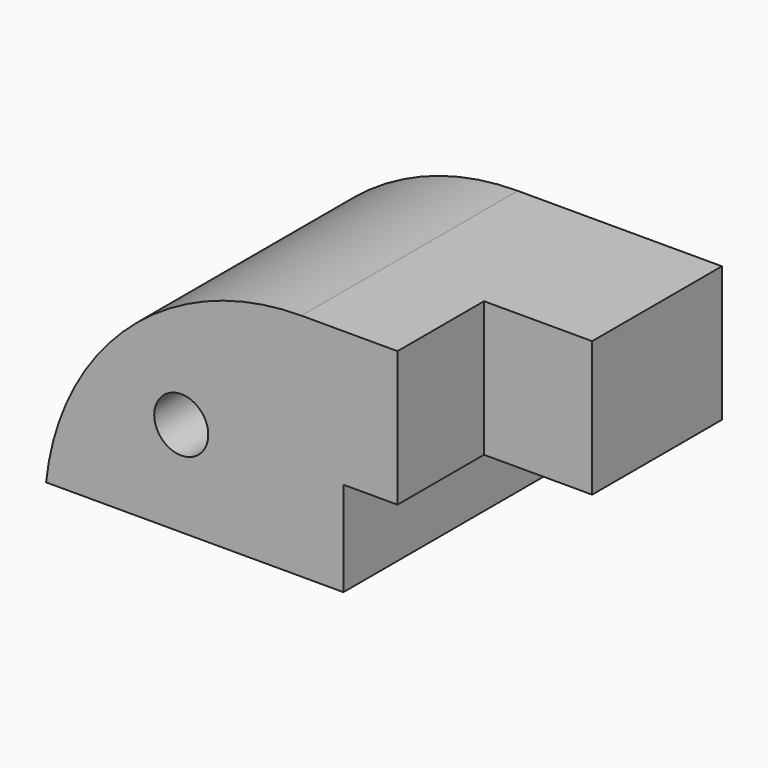
from build123d import *

# Parameters (mm, degrees)
F0_W         = 215.9
F0_H         = 127
F1_DEPTH     = 82.55
F2_W         = 76.2
F2_H         = 44.45
F3_DEPTH     = 127.001
F4_W         = 50.8
F4_H         = 37.5581905246
F5_DEPTH     = 82.551
F6_R         = 7.8160058593
F7_DEPTH     = 0.254
F8_R         = 12.7
F9_DEPTH     = 127.001
F10_T1_DEPTH = 699.3812649799
F11_DEPTH    = 107.95
F14_W        = 76.2
F14_H        = 44.45
F15_DEPTH    = 127.001
F13_W        = 50.8
F13_H        = 63.5
F16_DEPTH    = 50.8
F17_R        = 12.7
F18_DEPTH    = 127.001
F19_T1_DEPTH = 726.8985851792


# Not quite as in the source:
# - a fillet or chamfer that OpenCascade refuses, or shapes differently, is made with other operations: its cross-section is extruded or revolved along the edge and cut away or added


with BuildPart() as f1:
    # F0 (on Top) → F1 (new body)
    with BuildSketch(Plane.XY):
        with Locations((13.1497114167, 63.5)):
            Rectangle(F0_W, F0_H)
    extrude(amount=F1_DEPTH)

    # F2 (on face) → F3 (cut, through all)
    with BuildSketch(Plane(origin=(0, 127, 0), x_dir=(-1, 0, 0), z_dir=(0, 1, 0))):
        with Locations((-82.9997114167, 22.225)):
            Rectangle(F2_W, F2_H)
    extrude(amount=-F3_DEPTH, mode=Mode.SUBTRACT)

    # F4 (on face) → F5 (cut, through all)
    with BuildSketch(Plane.XY.offset(82.55)):
        with Locations((95.6997114167, 18.7790952623)):
            Rectangle(F4_W, F4_H)
    extrude(amount=-F5_DEPTH, mode=Mode.SUBTRACT)

    # F6 (on face) → F7 (cut)
    with BuildSketch(Plane.YZ.offset(121.0997114167)):
        with Locations((84.554515779, 63.2054284215)):
            Circle(F6_R)
    extrude(amount=-F7_DEPTH, mode=Mode.SUBTRACT)

    # F8 (on face) → F9 (cut, through all)
    with BuildSketch(Plane(origin=(0, 127, 0), x_dir=(-1, 0, 0), z_dir=(0, 1, 0))):
        with Locations((31.3002885833, 44.45)):
            Circle(F8_R)
    extrude(amount=-F9_DEPTH, mode=Mode.SUBTRACT)

    # F10: fillet of radius 120.65 on 1 edges, made by hand

    # F10_s2 → F10_t1 (cut)
    with BuildSketch(Plane.XZ.offset(-413.19063249)):
        with BuildLine():
            ThreePointArc((-94.8002885833, 0), (-50.8919372849, 59.7600722971), (19.6759644126, 82.55))
            Line((19.6759644126, 82.55), (19.6759644126, 84.963))
            Line((19.6759644126, 84.963), (-94.8002885833, 84.963))
            Line((-94.8002885833, 84.963), (-97.2132885833, 82.55))
            ThreePointArc((-97.2132885833, 82.55), (-97.2132885833, 41.275), (-97.0898136433, 0.762))
            Line((-97.0898136433, 0.762), (-94.8002885833, 0))
        make_face()
    extrude(amount=F10_T1_DEPTH, mode=Mode.SUBTRACT)

    # F0 (on Top) → F11 (join)
    with BuildSketch(Plane.XY):
        with Locations((13.1497114167, 63.5)):
            Rectangle(F0_W, F0_H)
    extrude(amount=F11_DEPTH)

    # F14 (on face) → F15 (cut, through all)
    with BuildSketch(Plane(origin=(0, 127, 0), x_dir=(-1, 0, 0), z_dir=(0, 1, 0))):
        with Locations((-82.9997114167, 22.225)):
            Rectangle(F14_W, F14_H)
    extrude(amount=-F15_DEPTH, mode=Mode.SUBTRACT)

    # F13 (on face) → F16 (cut)
    with BuildSketch(Plane.YZ.offset(121.0997114167)):
        with Locations((25.4, 76.2)):
            Rectangle(F13_W, F13_H)
    extrude(amount=-F16_DEPTH, mode=Mode.SUBTRACT)

    # F17 (on face) → F18 (cut, through all)
    with BuildSketch(Plane(origin=(0, 127, 0), x_dir=(-1, 0, 0), z_dir=(0, 1, 0))):
        with Locations((31.3002885833, 44.45)):
            Circle(F17_R)
    extrude(amount=-F18_DEPTH, mode=Mode.SUBTRACT)

    # F19: fillet of radius 120.65 on 1 edges, made by hand

    # F19_s2 → F19_t1 (cut)
    with BuildSketch(Plane.XZ.offset(-426.9492925896)):
        with BuildLine():
            ThreePointArc((-94.8002885833, 0), (-55.5180544698, 76.9902377631), (25.1794284525, 107.95))
            Line((25.1794284525, 107.95), (-94.8002885833, 107.95))
            Line((-94.8002885833, 107.95), (-94.8002885833, 0))
        make_face()
    extrude(amount=F19_T1_DEPTH, mode=Mode.SUBTRACT)


solid = f1.part
